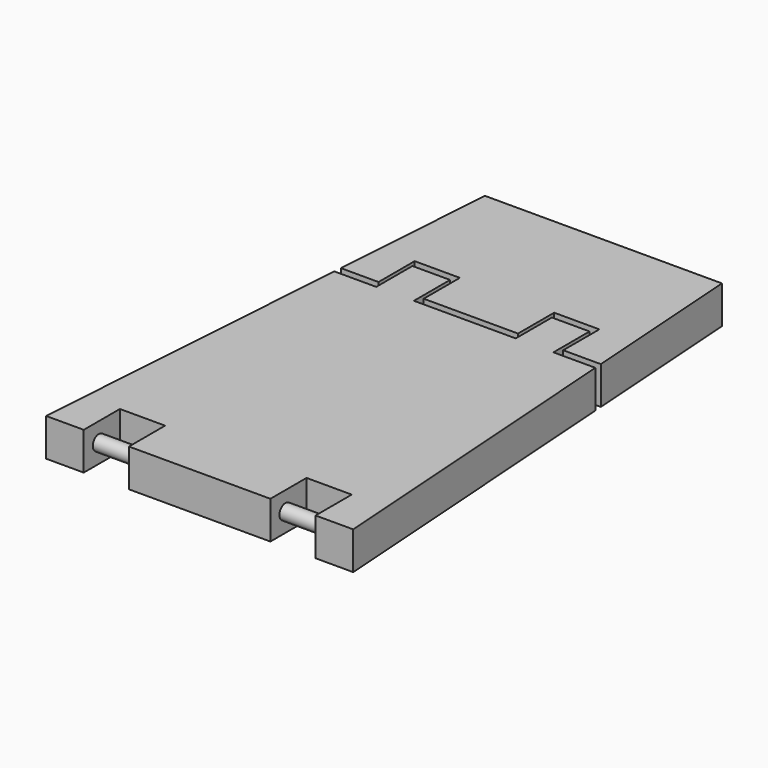
from build123d import *

# Parameters (mm, degrees)
F1_DEPTH = 5
F4_START = -6
F3_R     = 1.5
F3_R_2   = 1
F4_DEPTH = 28.8
F5_START = -5.4
F5_DEPTH = 30.3
F8_START = -10.4
F7_R     = 1
F8_DEPTH = 37.1


# Not quite as in the source:
# - a feature names something its author has since deleted; it is built from what else it names


with BuildPart() as f1:
    # F0 (on Top) → F1 (new body)
    with BuildSketch(Plane.XY):
        Polygon((-15.7285978556, -106.966223469), (-17.2584383383, -128.966223469), (-12.2584383383, -128.966223469), (-12.2584383383, -122.966223469), (-6.2584383383, -122.966223469), (-6.2584383383, -128.966223469), (6.2584383383, -128.966223469), (6.2584383383, -122.966223469), (12.2584383383, -122.966223469), (12.2584383383, -128.966223469), (17.2584383383, -128.966223469), (15.7285978556, -106.966223469), align=None)
    extrude(amount=F1_DEPTH)



with BuildPart() as f1b:
    # F0 (on Top) → F1, piece 2 (new body)
    with BuildSketch(Plane.XY):
        Polygon((-17.3279765421, -129.966223469), (-20.3876575074, -173.966223469), (-15.3876575074, -173.966223469), (-15.3876575074, -167.966223469), (-9.3876575074, -167.966223469), (-9.3876575074, -173.966223469), (9.3876575074, -173.966223469), (9.3876575074, -167.966223469), (15.3876575074, -167.966223469), (15.3876575074, -173.966223469), (20.3876575074, -173.966223469), (17.3279765421, -129.966223469), (11.7584383383, -129.966223469), (11.7584383383, -123.966223469), (6.7584383383, -123.966223469), (6.7584383383, -129.966223469), (-6.7584383383, -129.966223469), (-6.7584383383, -123.966223469), (-11.7584383383, -123.966223469), (-11.7584383383, -129.966223469), align=None)
    extrude(amount=F1_DEPTH)

    # F3 (on offset) → F4 (cut)
    with BuildSketch(Plane.YZ.offset(21.7584383383).offset(F4_START)):
        with Locations((-126.466223469, 2.5)):
            Circle(F3_R)
        with Locations((-126.466223469, 2.5)):
            Circle(F3_R_2, mode=Mode.SUBTRACT)
    extrude(amount=-F4_DEPTH, mode=Mode.SUBTRACT)


with BuildPart() as f1_1:
    add(f1.part)

    add(f1b.part)  # F5 merges F1b
    # F3 (on offset) → F5 (join)
    with BuildSketch(Plane.YZ.offset(21.7584383383).offset(F5_START)):
        with Locations((-126.466223469, 2.5)):
            Circle(F3_R_2)
    extrude(amount=-F5_DEPTH)

    # F7 (on offset) → F8 (join)
    with BuildSketch(Plane.YZ.offset(29.3876575074).offset(F8_START)):
        with Locations((-171.466223469, 2.5)):
            Circle(F7_R)
    extrude(amount=-F8_DEPTH)


solid = f1_1.part
